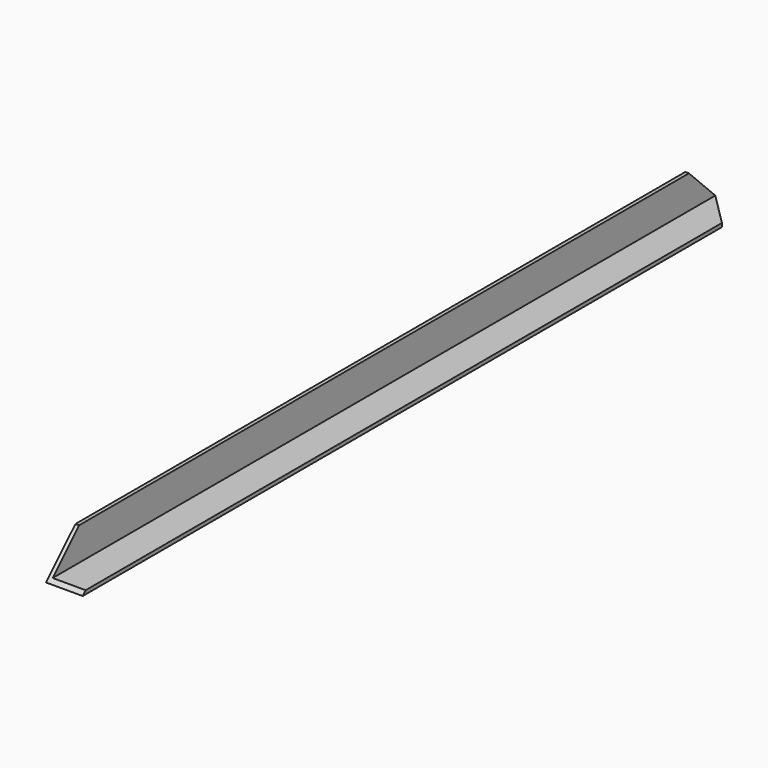
from build123d import *

# Parameters (mm, degrees)
F1_DEPTH = 570
F3_DEPTH = 50
F5_DEPTH = 50


# Not quite as in the source:
# - a feature names something its author has since deleted; it is built from what else it names


with BuildPart() as f1:
    # F0 (on Front) → F1 (new body, symmetric)
    with BuildSketch(Plane.XZ):
        Polygon((0, 50), (0, 0), (50, 0), (50, 5), (5, 5), (5, 50), align=None)
    extrude(amount=F1_DEPTH, both=True)

    # F2 (on face) → F3 (cut)
    with BuildSketch(Plane(origin=(0, 0, 0), x_dir=(0, -1, 0), z_dir=(-1, 0, 0))):
        Polygon((-570, 50), (-570, 0), (-520, 50), align=None)
        Polygon((520, 50), (570, 0), (570, 50), align=None)
    extrude(amount=-F3_DEPTH, mode=Mode.SUBTRACT)

    # F4 (on face) → F5 (cut)
    with BuildSketch(Plane(origin=(0, 0, 0), x_dir=(1, 0, 0), z_dir=(0, 0, -1))):
        Polygon((50, -520), (0, -570), (50, -570), align=None)
    extrude(amount=-F5_DEPTH, mode=Mode.SUBTRACT)


solid = f1.part
